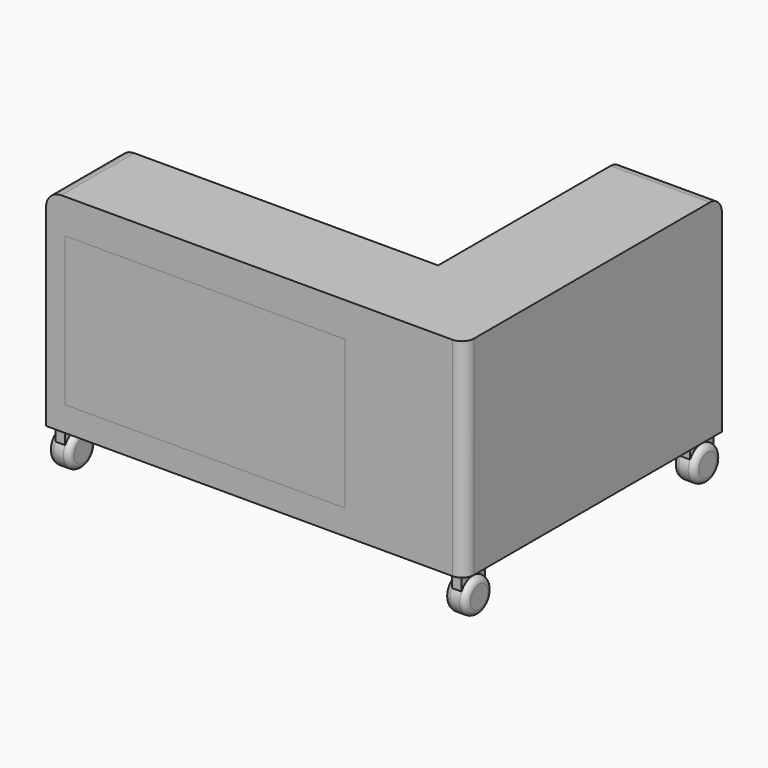
from build123d import *

# Parameters (mm, degrees)
F1_DEPTH  = 38.27951
F2_W      = 117.4374558032
F2_H      = 62.3886492103
F3_DEPTH  = 38.28051
F4_W      = 117.4374558032
F4_H      = 62.3886492103
F5_DEPTH  = 2
F6_W      = 117.4374558032
F6_H      = 49.5720207691
F7_DEPTH  = 2
F8_W      = 117.4374558032
F8_H      = 12.8166284412
F9_DEPTH  = 2
F11_W     = 8
F11_H     = 7
F12_DEPTH = 1.5
F14_DEPTH = 1.5
F17_DEPTH = 41.64187
F18_R     = 5
F19_W     = 78.5573190078
F19_H     = 70.0646340847
F20_DEPTH = 39
F22_DEPTH = 37
F21_W     = 78.5573190078
F21_H     = 2
F23_W     = 78.5573190078
F23_H     = 70.0646340847
F24_DEPTH = 1.71646
F25_W     = 6.4101852477
F25_H     = 10.5219734833
F26_DEPTH = 1
F27_R     = 7.139328944
F28_DEPTH = 9
F29_R     = 2.5
F32_DEPTH = 4


with BuildPart() as f1:
    # F0 (on Front) → F1 (new body)
    with BuildSketch(Plane.XZ):
        with BuildLine():
            Line((66.9957697392, 49.2157749832), (-60.6457697392, 49.2157749832))
            ThreePointArc((-60.6457697392, 49.2157749832), (-65.1358977997, 47.3559030437), (-66.9957697392, 42.8657749832))
            Line((-66.9957697392, 42.8657749832), (-66.9957697392, -38.1549037993))
            Line((-66.9957697392, -38.1549037993), (66.9957697392, -38.1549037993))
            Line((66.9957697392, -38.1549037993), (66.9957697392, 49.2157749832))
        make_face()
    extrude(amount=F1_DEPTH)

    # F2 (on face) → F3 (cut, through all)
    with BuildSketch(Plane.XZ.offset(38.27951)):
        with Locations((-0.2467352897, 3.4934589639)):
            Rectangle(F2_W, F2_H)
    extrude(amount=-F3_DEPTH, mode=Mode.SUBTRACT)


with BuildPart() as f5:
    # F4 (on face) → F5 (new body)
    with BuildSketch(Plane.XZ.offset(38.27951)):
        with Locations((-0.2467352897, 3.4934589639)):
            Rectangle(F4_W, F4_H)
    extrude(amount=-F5_DEPTH)


with BuildPart() as f7:
    # F6 (on face) → F7 (new body)
    with BuildSketch(Plane(origin=(0, 0, 0), x_dir=(-1, 0, 0), z_dir=(0, 1, 0))):
        with Locations((0.2467352897, -2.9148552567)):
            Rectangle(F6_W, F6_H)
    extrude(amount=-F7_DEPTH)


with BuildPart() as f9:
    # F8 (on face) → F9 (new body)
    with BuildSketch(Plane(origin=(0, 0, 0), x_dir=(-1, 0, 0), z_dir=(0, 1, 0))):
        with Locations((0.2467352897, 28.2794693485)):
            Rectangle(F8_W, F8_H)
    extrude(amount=-F9_DEPTH)


with BuildPart() as f12_tool:
    # F11 (on offset) → F12 (new body)
    with BuildSketch(Plane(origin=(0, 0, 0), x_dir=(-1, 0, 0), z_dir=(0, 1, 0))):
        with Locations((-33.4628044665, 34.19829382)):
            Rectangle(F11_W, F11_H)
        with Locations((24.7542907447, 34.19829382)):
            Rectangle(F11_W, F11_H)
    extrude(amount=-F12_DEPTH)


with BuildPart() as f1_1:
    add(f1.part)

    # F12: cut by f12_tool
    add(f12_tool.part, mode=Mode.SUBTRACT)

    # F16 (on offset) → F17 (join)
    with BuildSketch(Plane.YZ.offset(66.9957697392)):
        with BuildLine():
            Line((0, 49.2157749832), (-38.27951, 49.2157749832))
            Line((-38.27951, 49.2157749832), (-38.27951, -38.1549037993))
            Line((-38.27951, -38.1549037993), (0, -38.1549037993))
            Line((0, -38.1549037993), (96.9052836299, -38.1549037993))
            Line((96.9052836299, -38.1549037993), (96.9052836299, 42.8657749832))
            ThreePointArc((96.9052836299, 42.8657749832), (95.0454116904, 47.3559030437), (90.5552836299, 49.2157749832))
            Line((90.5552836299, 49.2157749832), (0, 49.2157749832))
        make_face()
    extrude(amount=F17_DEPTH)

    # F18
    f18_edges = [f1_1.edges().sort_by_distance(p)[0] for p in [
        (108.63764, -38.27951, 5.530436),
    ]]
    fillet(f18_edges, radius=F18_R)

    # F19 (on face) → F20 (cut)
    with BuildSketch(Plane(origin=(66.9957697392, 0, 0), x_dir=(0, -1, 0), z_dir=(-1, 0, 0))):
        with Locations((-48.2019898482, 4.7012194991)):
            Rectangle(F19_W, F19_H)
    extrude(amount=-F20_DEPTH, mode=Mode.SUBTRACT)


with BuildPart() as f9_1:
    add(f9.part)

    # F12: cut by f12_tool
    add(f12_tool.part, mode=Mode.SUBTRACT)


with BuildPart() as f14:
    # F13 (on offset) → F14 (new body)
    with BuildSketch(Plane(origin=(0, 0, 0), x_dir=(-1, 0, 0), z_dir=(0, 1, 0))):
        Polygon((-29.4628044665, 37.69829382), (-37.4628044665, 37.69829382), (-37.4628044665, 34.6877835691), (-37.4628044665, 30.69829382), (-29.4628044665, 30.69829382), (-29.4628044665, 34.6877835691), align=None)
    extrude(amount=-F14_DEPTH)


with BuildPart() as f14b:
    # F13 (on offset) → F14, piece 2 (new body)
    with BuildSketch(Plane(origin=(0, 0, 0), x_dir=(-1, 0, 0), z_dir=(0, 1, 0))):
        Polygon((28.7542907447, 37.69829382), (20.7542907447, 37.69829382), (20.7542907447, 34.6877835691), (20.7542907447, 30.69829382), (28.7542907447, 30.69829382), (28.7542907447, 34.6877835691), align=None)
    extrude(amount=-F14_DEPTH)


with BuildPart() as f22:
    # F21 (on face) → F22 (new body)
    with BuildSketch(Plane(origin=(105.9957697392, 0, 0), x_dir=(0, -1, 0), z_dir=(-1, 0, 0))):
        Polygon((-87.4806493521, 16.8134574331), (-87.4806493521, 15.8134574331), (-8.9233303443, 15.8134574331), (-8.9233303443, 17.8134574331), (-87.4806493521, 17.8134574331), align=None)
    extrude(amount=F22_DEPTH)


with BuildPart() as f22b:
    # F21 (on face) → F22, piece 2 (new body)
    with BuildSketch(Plane(origin=(105.9957697392, 0, 0), x_dir=(0, -1, 0), z_dir=(-1, 0, 0))):
        with Locations((-48.2019898482, -6.1865425669)):
            Rectangle(F21_W, F21_H)
    extrude(amount=F22_DEPTH)


with BuildPart() as f24:
    # F23 (on face) → F24 (new body)
    with BuildSketch(Plane(origin=(66.9957697392, 0, 0), x_dir=(0, -1, 0), z_dir=(-1, 0, 0))):
        with Locations((-48.2019898482, 4.7012194991)):
            Rectangle(F23_W, F23_H)
    extrude(amount=-F24_DEPTH)

    # F25 (on face) → F26 (join)
    with BuildSketch(Plane(origin=(66.9957697392, 0, 0), x_dir=(0, -1, 0), z_dir=(-1, 0, 0))):
        with Locations((-24.0586362779, 5.2609867416)):
            Rectangle(F25_W, F25_H)
    extrude(amount=F26_DEPTH)


with BuildPart() as f28:
    # F27 (on face) → F28 (new body)
    with BuildSketch(Plane.YZ.offset(108.6376397392)):
        with Locations((89.475736022, -47.3454110324)):
            Circle(F27_R)
    extrude(amount=-F28_DEPTH)

    # F29
    f29_edges = [f28.edges().sort_by_distance(p)[0] for p in [
        (108.63764, 82.336407, -47.345411),
        (99.63764, 82.336407, -47.345411),
    ]]
    fillet(f29_edges, radius=F29_R)

    # F31 (on offset) → F32 (join)
    with BuildSketch(Plane.YZ.offset(106.1376397392)):
        with BuildLine():
            ThreePointArc((83.319671452, -43.7297663068), (89.475736022, -40.2060820884), (95.6318005919, -43.7297663068))
            Line((95.6318005919, -43.7297663068), (95.6318005919, -38.1549037993))
            Line((95.6318005919, -38.1549037993), (83.319671452, -38.1549037993))
            Line((83.319671452, -38.1549037993), (83.319671452, -43.7297663068))
        make_face()
    extrude(amount=-F32_DEPTH)


with BuildPart() as f35_1:
    # F35: instance of F28
    add(f28.part.mirror(Plane.YZ.offset(87.8167047392)))


with BuildPart() as f36_1:
    # F36: copy of F28
    add(f28.part.moved(Location((0, -119.9988, 0))))


with BuildPart() as f37_1:
    # F37: copy of F36_1
    add(f36_1.part.moved(Location((-166.40481, 0, 0))))


with BuildPart() as f40_1:
    # F40: instance of F37_1
    add(f37_1.part.mirror(Plane(origin=(0, -19.139755, 0), x_dir=(-1, 0, 0), z_dir=(0, 1, 0))))


with BuildPart() as f41_1:
    # F41: copy of F40_1
    add(f40_1.part.moved(Location((133.58488, 7.02052, 0))))


solid = Compound([f5.part, f7.part, f1_1.part, f9_1.part, f14.part, f14b.part, f22.part, f22b.part, f24.part, f28.part, f35_1.part, f36_1.part, f37_1.part, f40_1.part, f41_1.part])
